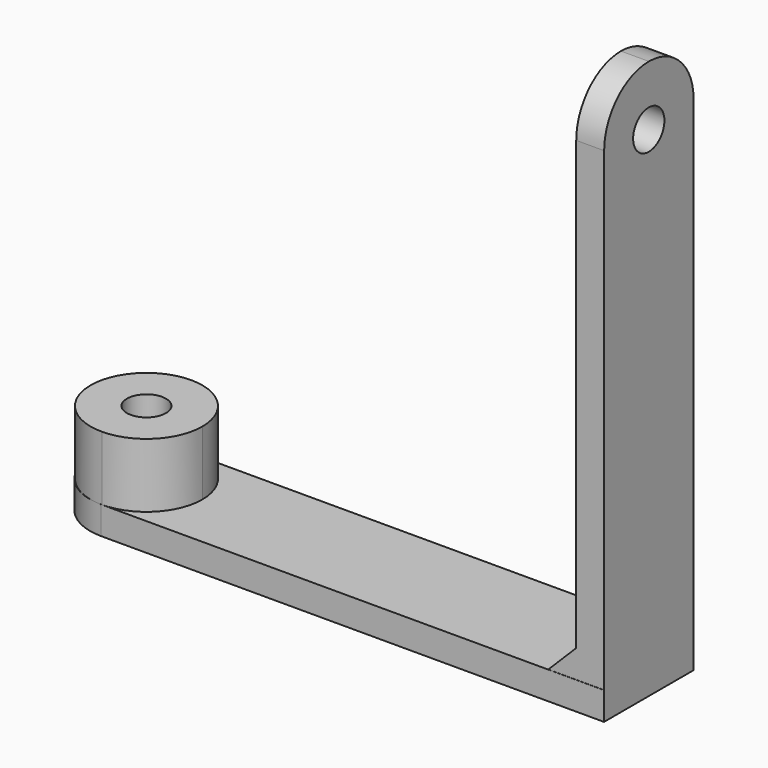
from build123d import *

# Parameters (mm, degrees)
F0_R     = 3.5
F1_DEPTH = 5
F2_R     = 9.99999
F4_START = 5
F3_W     = 5
F3_H     = 20
F4_DEPTH = 95
F5_R     = 3.5
F6_DEPTH = 79.3
F7_R     = 9.99999
F8_DEPTH = 16.5
F3_W_2   = 7
F9_DEPTH = 10
F10_SIZE = 6.99999


# Not quite as in the source:
# - a fillet or chamfer is up to 0.001 mm smaller than in the source, because OpenCascade refuses the exact size


with BuildPart() as f1:
    # F0 (on Top) → F1 (new body)
    with BuildSketch(Plane.XY):
        with BuildLine():
            Line((-36.1016022205, 30.0462352857), (-46.2016022205, 30.0462352857))
            Line((-46.2016022205, 30.0462352857), (-46.2016022205, 10.0462352857))
            Line((-46.2016022205, 10.0462352857), (-36.1016022205, 10.0462352857))
            ThreePointArc((-36.1016022205, 10.0462352857), (-46.1016022205, 20.0462352857), (-36.1016022205, 30.0462352857))
        make_face()
        with BuildLine():
            Line((53.7983977795, 30.0462352857), (-36.1016022205, 30.0462352857))
            ThreePointArc((-36.1016022205, 30.0462352857), (-29.0305344087, 27.1173030976), (-26.1016022205, 20.0462352857))
            ThreePointArc((-26.1016022205, 20.0462352857), (-29.0305344087, 12.9751674738), (-36.1016022205, 10.0462352857))
            Line((-36.1016022205, 10.0462352857), (53.7983977795, 10.0462352857))
            Line((53.7983977795, 10.0462352857), (53.7983977795, 30.0462352857))
        make_face()
        with BuildLine():
            ThreePointArc((-26.1016022205, 20.0462352857), (-29.0305344087, 27.1173030976), (-36.1016022205, 30.0462352857))
            ThreePointArc((-36.1016022205, 30.0462352857), (-46.1016022205, 20.0462352857), (-36.1016022205, 10.0462352857))
            ThreePointArc((-36.1016022205, 10.0462352857), (-29.0305344087, 12.9751674738), (-26.1016022205, 20.0462352857))
        make_face()
        with Locations((-36.1016022205, 20.0462352857)):
            Circle(F0_R, mode=Mode.SUBTRACT)
    extrude(amount=F1_DEPTH)

    # F2 (radius 10 in the source; OpenCascade refuses exactly that, so slightly less here)
    f2_edges = [f1.edges().sort_by_distance(p)[0] for p in [
        (-46.201602, 30.046235, 2.5),
        (-46.201602, 10.046235, 2.5),
    ]]
    fillet(f2_edges, radius=F2_R)

    # F3 (on Top) → F4 (join)
    with BuildSketch(Plane.XY.offset(F4_START)):
        with Locations((51.2983977795, 20.0760087371)):
            Rectangle(F3_W, F3_H)
    extrude(amount=F4_DEPTH)

    # F5 (on Right) → F6 (cut)
    with BuildSketch(Plane.YZ):
        with Locations((20.0534593314, 89.2638255358)):
            Circle(F5_R)
    extrude(amount=F6_DEPTH, mode=Mode.SUBTRACT)

    # F7 (radius 10 in the source; OpenCascade refuses exactly that, so slightly less here)
    f7_edges = [f1.edges().sort_by_distance(p)[0] for p in [
        (51.298398, 10.076009, 100),
        (51.298398, 30.076009, 100),
    ]]
    fillet(f7_edges, radius=F7_R)

    # F0 (on Top) → F8 (join)
    with BuildSketch(Plane.XY):
        with BuildLine():
            ThreePointArc((-26.1016022205, 20.0462352857), (-29.0305344087, 27.1173030976), (-36.1016022205, 30.0462352857))
            ThreePointArc((-36.1016022205, 30.0462352857), (-46.1016022205, 20.0462352857), (-36.1016022205, 10.0462352857))
            ThreePointArc((-36.1016022205, 10.0462352857), (-29.0305344087, 12.9751674738), (-26.1016022205, 20.0462352857))
        make_face()
        with Locations((-36.1016022205, 20.0462352857)):
            Circle(F0_R, mode=Mode.SUBTRACT)
    extrude(amount=F8_DEPTH)

    # F3 (on Top) → F9 (join)
    with BuildSketch(Plane.XY):
        with Locations((51.2983977795, 20.0760087371)):
            Rectangle(F3_W, F3_H)
        with Locations((45.2983977795, 20.0760087371)):
            Rectangle(F3_W_2, F3_H)
    extrude(amount=F9_DEPTH)

    # F10 (size 7 in the source; OpenCascade refuses exactly that, so slightly less here)
    f10_edges = [f1.edges().sort_by_distance(p)[0] for p in [
        (41.798398, 20.076009, 10),
    ]]
    chamfer(f10_edges, length=F10_SIZE)


solid = f1.part
